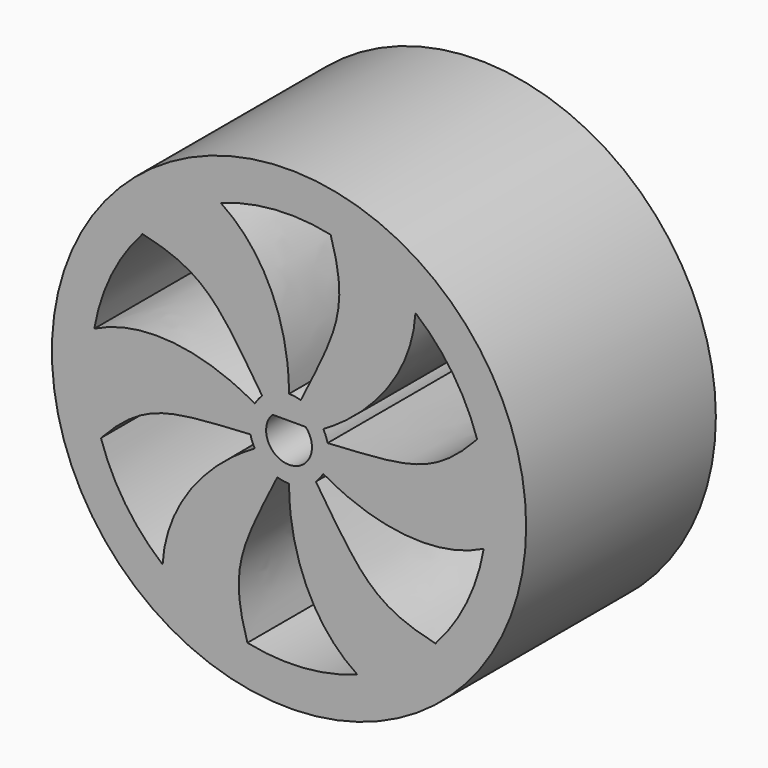
from build123d import *

# Parameters (mm, degrees)
F0_R            = 15
F1_DEPTH        = 15
F3_DEPTH        = 5.5
F5_DEPTH        = 15.001
F5_COPIES_COUNT = 6


# Not quite as in the source:
# - a pattern or mirror of a feature is missing from the dataset's text; its kind, count and spacing are read off the source's solid


with BuildPart() as f1:
    # F0 (on Front) → F1 (new body)
    with BuildSketch(Plane.XZ):
        Circle(F0_R)
    extrude(amount=-F1_DEPTH)

    # F2 (on face) → F3 (cut)
    with BuildSketch(Plane.XZ):
        with BuildLine():
            ThreePointArc((-1.0499999991, 1.000000001), (-0.5385164813, -1.3462912015), (1.45, 0))
            ThreePointArc((1.45, 0), (1.3462912015, 0.5385164813), (1.0499999991, 1.000000001))
            Line((1.0499999991, 1.000000001), (-1.0499999991, 1.000000001))
        make_face()
    extrude(amount=-F3_DEPTH, mode=Mode.SUBTRACT)

    # F4 (on face) → F5 (cut, through all)
    with BuildSketch(Plane.XZ):
        with BuildLine():
            ThreePointArc((2.6320639833, 12.2197479183), (-0.8786691083, 12.4690793805), (-4.3197418021, 11.7298691708))
            add(Edge.make_bspline(
                [(-4.3197418021, 11.7298691708), (-1.5711041633, 9.9351070821), (0, 6.4156376757), (0, 2.5)],
                knots=[0, 0, 0, 0, 10.1907141136, 10.1907141136, 10.1907141136, 10.1907141136], degree=3))
            ThreePointArc((0, 2.5), (0.3749457354, 2.4717232239), (0.7414096655, 2.3875325564))
            add(Edge.make_bspline(
                [(2.6320639833, 12.2197479183), (3.8345751818, 8.3321332932), (2.9968102463, 6.907931529), (0.7414096655, 2.3875325564)],
                knots=[0, 0, 0, 0, 10.0123440149, 10.0123440149, 10.0123440149, 10.0123440149], degree=3))
        make_face()
    f5 = extrude(amount=-F5_DEPTH, mode=Mode.SUBTRACT)

    # F5_copies: F5 ×6 about axis
    f5_copies_axis = Axis((0, 0, 0), (0, 1, 0))
    for i in range(1, F5_COPIES_COUNT):
        add(f5.rotate(f5_copies_axis, i * 360 / F5_COPIES_COUNT), mode=Mode.SUBTRACT)


solid = f1.part
